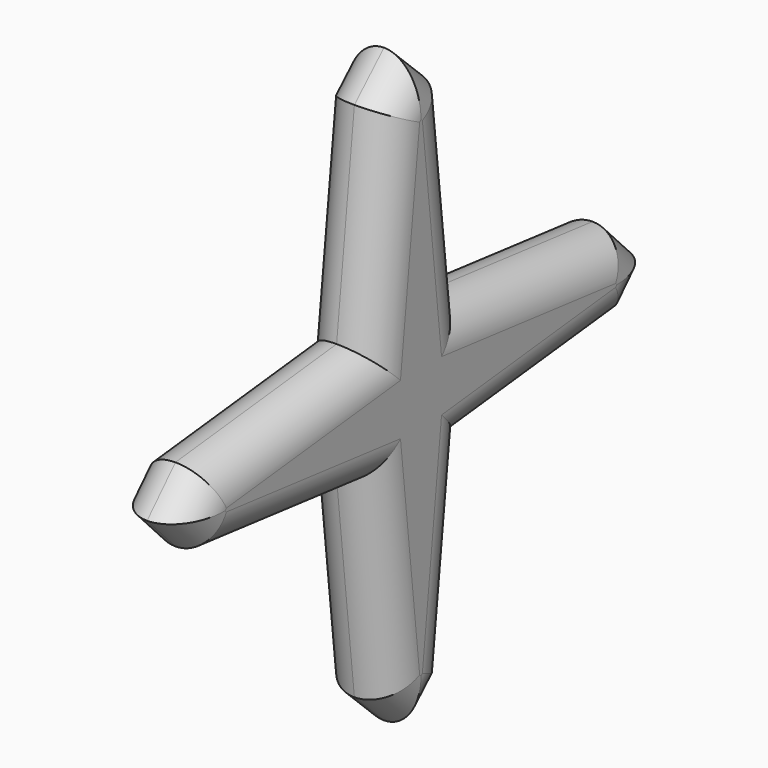
from build123d import *

# Parameters (mm, degrees)
F1_DEPTH = 3.175
F2_R     = 3.17499


# Not quite as in the source:
# - a fillet or chamfer is up to 0.001 mm smaller than in the source, because OpenCascade refuses the exact size


with BuildPart() as f1:
    # F0 (on Right) → F1 (new body, symmetric)
    with BuildSketch(Plane.YZ):
        Polygon((3.175, 22.364773135), (0, 25.4), (-3.175, 22.364773135), (-5.08, 5.08), (-22.364773135, 3.175), (-25.4, 0), (-22.364773135, -3.175), (-5.08, -5.08), (-3.175, -22.364773135), (0, -25.4), (3.175, -22.364773135), (5.08, -5.08), (22.364773135, -3.175), (25.4, 0), (22.364773135, 3.175), (5.08, 5.08), align=None)
    extrude(amount=F1_DEPTH, both=True)

    # F2 (radius 3.175 in the source; OpenCascade refuses exactly that, so slightly less here)
    f2_edges = [f1.edges().sort_by_distance(p)[0] for p in [
        (3.175, 4.1275, 13.722387),
        (3.175, 1.5875, 23.882387),
        (3.175, -1.5875, 23.882387),
        (3.175, -4.1275, 13.722387),
        (3.175, -13.722387, 4.1275),
        (3.175, -23.882387, 1.5875),
        (3.175, -23.882387, -1.5875),
        (3.175, -13.722387, -4.1275),
        (3.175, -4.1275, -13.722387),
        (3.175, -1.5875, -23.882387),
        (3.175, 1.5875, -23.882387),
        (3.175, 4.1275, -13.722387),
        (3.175, 13.722387, -4.1275),
        (3.175, 23.882387, -1.5875),
        (3.175, 23.882387, 1.5875),
        (3.175, 13.722387, 4.1275),
        (-3.175, 4.1275, 13.722387),
        (-3.175, 1.5875, 23.882387),
        (-3.175, -1.5875, 23.882387),
        (-3.175, -4.1275, 13.722387),
        (-3.175, -13.722387, 4.1275),
        (-3.175, -23.882387, 1.5875),
        (-3.175, -23.882387, -1.5875),
        (-3.175, -13.722387, -4.1275),
        (-3.175, -4.1275, -13.722387),
        (-3.175, -1.5875, -23.882387),
        (-3.175, 1.5875, -23.882387),
        (-3.175, 4.1275, -13.722387),
        (-3.175, 13.722387, -4.1275),
        (-3.175, 23.882387, -1.5875),
        (-3.175, 23.882387, 1.5875),
        (-3.175, 13.722387, 4.1275),
    ]]
    fillet(f2_edges, radius=F2_R)


solid = f1.part
